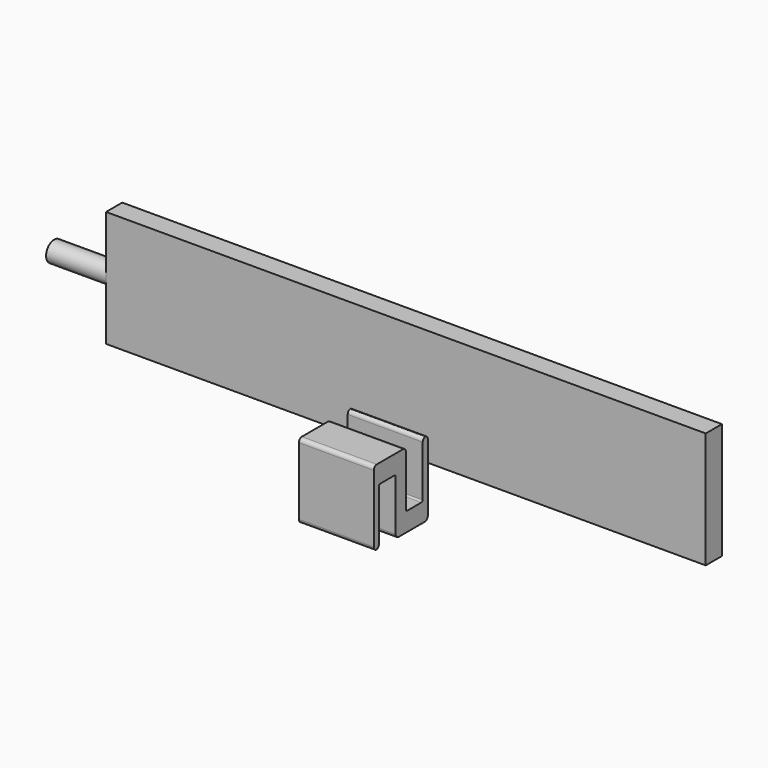
from build123d import *

# Parameters (mm, degrees)
F0_W        = 100
F0_H        = 100
F1_DEPTH    = 22.5
F2_W        = 28
F2_H        = 75
F3_DEPTH    = 100
F5_DEPTH    = 50
F6_T1_DEPTH = 125
F7_R        = 2
F8_W        = 27
F8_H        = 155
F9_DEPTH    = 400
F10_R       = 13.5
F11_DEPTH   = 80


# Not quite as in the source:
# - a fillet or chamfer that OpenCascade refuses, or shapes differently, is made with other operations: its cross-section is extruded or revolved along the edge and cut away or added


with BuildPart() as f1:
    # F0 (on Front) → F1 (new body, symmetric)
    with BuildSketch(Plane.XZ):
        Rectangle(F0_W, F0_H)
    extrude(amount=F1_DEPTH, both=True)

    # F2 (on face) → F3 (cut, symmetric)
    with BuildSketch(Plane.YZ.offset(50)):
        with Locations((0, 12.5)):
            Rectangle(F2_W, F2_H)
    extrude(amount=F3_DEPTH, both=True, mode=Mode.SUBTRACT)

    # F4 (on Right) → F5 (join, symmetric)
    with BuildSketch(Plane.YZ):
        Polygon((-22.5, -50), (-22.5, 50), (-67.5, 50), (-67.5, -50), (-59, -50), (-59, 25), (-31, 25), (-31, -50), align=None)
    extrude(amount=F5_DEPTH, both=True)

    # F6: fillet of radius 5 on 8 edges, made by hand

    # F6_s2 → F6_t1 (cut)
    with BuildSketch(Plane.YZ.offset(-62.5)):
        with BuildLine():
            ThreePointArc((-19, 50), (-15.4644660941, 48.5355339059), (-14, 45))
            Line((-14, 45), (-14, 50))
            Line((-14, 50), (-19, 50))
        make_face()
        with BuildLine():
            ThreePointArc((14, 45), (15.4644660941, 48.5355339059), (19, 50))
            Line((19, 50), (14, 50))
            Line((14, 50), (14, 45))
        make_face()
        with BuildLine():
            ThreePointArc((-59, -45), (-60.4644660941, -48.5355339059), (-64, -50))
            Line((-64, -50), (-59, -50))
            Line((-59, -50), (-59, -45))
        make_face()
        with BuildLine():
            ThreePointArc((-67.5, 45), (-66.0355339059, 48.5355339059), (-62.5, 50))
            Line((-62.5, 50), (-67.5, 50))
            Line((-67.5, 50), (-67.5, 45))
        make_face()
        with BuildLine():
            ThreePointArc((-62.5, -50), (-66.0355339059, -48.5355339059), (-67.5, -45))
            Line((-67.5, -45), (-67.5, -50))
            Line((-67.5, -50), (-62.5, -50))
        make_face()
        with BuildLine():
            ThreePointArc((17.5, 50), (21.0355339059, 48.5355339059), (22.5, 45))
            Line((22.5, 45), (22.5, 50))
            Line((22.5, 50), (17.5, 50))
        make_face()
        with BuildLine():
            ThreePointArc((-26, -50), (-29.5355339059, -48.5355339059), (-31, -45))
            Line((-31, -45), (-31, -50))
            Line((-31, -50), (-26, -50))
        make_face()
        with BuildLine():
            ThreePointArc((17.5, -50), (21.0355339059, -48.5355339059), (22.5, -45))
            Line((22.5, -45), (22.5, -50))
            Line((22.5, -50), (17.5, -50))
        make_face()
    extrude(amount=F6_T1_DEPTH, mode=Mode.SUBTRACT)

    # F7
    f7_edges = [f1.edges().sort_by_distance(p)[0] for p in [
        (0, 14, -25),
        (0, -14, -25),
        (0, -31, 25),
        (0, -59, 25),
    ]]
    fillet(f7_edges, radius=F7_R)


with BuildPart() as f9:
    # F8 (on Right) → F9 (new body, symmetric)
    with BuildSketch(Plane.YZ):
        with Locations((61.9791960033, 77.5)):
            Rectangle(F8_W, F8_H)
    extrude(amount=F9_DEPTH, both=True)

    # F10 (on face) → F11 (join)
    with BuildSketch(Plane(origin=(-400, 0, 0), x_dir=(0, -1, 0), z_dir=(-1, 0, 0))):
        with Locations((-61.9791960033, 77.5)):
            Circle(F10_R)
    extrude(amount=F11_DEPTH)


solid = Compound([f1.part, f9.part])
